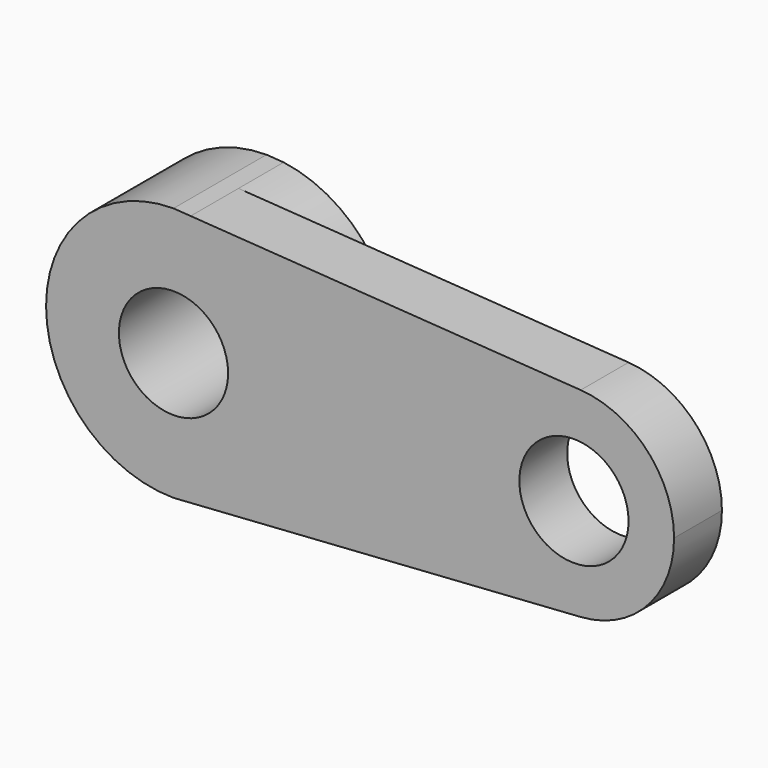
from build123d import *

# Parameters (mm, degrees)
F0_R     = 19.05
F1_DEPTH = 20.8662841469
F2_DEPTH = 40.5588373542


# Not quite as in the source:
# - the program builds the solid bodies; features that only make, move or delete a surface that nothing else refers to are left out


with BuildPart() as f1:
    # F0 (on Front) → F1 (new body)
    with BuildSketch(Plane.XZ):
        with BuildLine():
            Line((5.983272408, 44.0454645939), (0, 44.45))
            ThreePointArc((0, 44.45), (-44.45, 0), (0, -44.45))
            Line((0, -44.45), (5.983272408, -44.0454645939))
            ThreePointArc((5.983272408, -44.0454645939), (33.4795382177, -29.2390666871), (44.45, 0))
            ThreePointArc((44.45, 0), (33.4795382177, 29.2390666871), (5.983272408, 44.0454645939))
        make_face()
        Circle(F0_R, mode=Mode.SUBTRACT)
        with BuildLine():
            Line((142.0559377087, 34.8454470844), (5.983272408, 44.0454645939))
            ThreePointArc((5.983272408, 44.0454645939), (33.4795382177, 29.2390666871), (44.45, 0))
            ThreePointArc((44.45, 0), (33.4795382177, -29.2390666871), (5.983272408, -44.0454645939))
            Line((5.983272408, -44.0454645939), (142.0559377087, -34.8454470844))
            ThreePointArc((142.0559377087, -34.8454470844), (104.775, 0), (142.0559377087, 34.8454470844))
        make_face()
        with BuildLine():
            ThreePointArc((174.625, 0), (165.2150617232, 23.8482127268), (142.0559377087, 34.8454470844))
            ThreePointArc((142.0559377087, 34.8454470844), (104.775, 0), (142.0559377087, -34.8454470844))
            ThreePointArc((142.0559377087, -34.8454470844), (165.2150617232, -23.8482127268), (174.625, 0))
        make_face()
        with Locations((139.7, 0)):
            Circle(F0_R, mode=Mode.SUBTRACT)
    extrude(amount=-F1_DEPTH)

    # F0 (on Front) → F2 (join)
    with BuildSketch(Plane.XZ):
        with BuildLine():
            Line((5.983272408, 44.0454645939), (0, 44.45))
            ThreePointArc((0, 44.45), (-44.45, 0), (0, -44.45))
            Line((0, -44.45), (5.983272408, -44.0454645939))
            ThreePointArc((5.983272408, -44.0454645939), (33.4795382177, -29.2390666871), (44.45, 0))
            ThreePointArc((44.45, 0), (33.4795382177, 29.2390666871), (5.983272408, 44.0454645939))
        make_face()
        Circle(F0_R, mode=Mode.SUBTRACT)
    extrude(amount=-F2_DEPTH)


solid = f1.part
